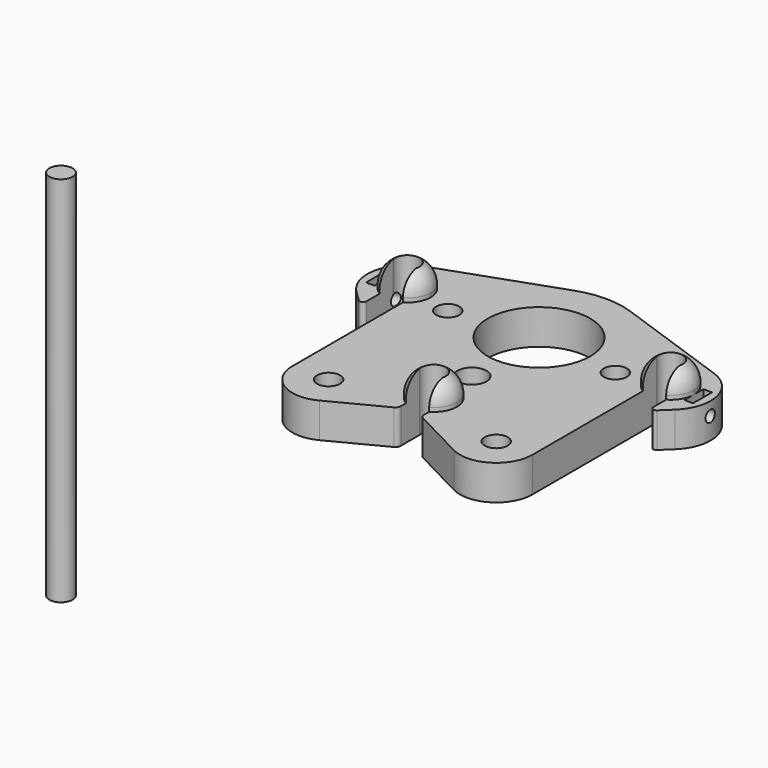
from build123d import *

# Parameters (mm, degrees)
F0_R        = 3.1496
F0_R_2      = 3.9624
F0_R_3      = 16.51
F1_DEPTH    = 9.525
F0_R_4      = 13.97
F2_DEPTH    = 9.525
F5_DEPTH    = 8.636
F6_T1_DEPTH = 2.3368
F6_T3_DEPTH = 2.3368
F7_DEPTH    = 6.35
F8_T2_ANGLE = 359.64
F8_T4_ANGLE = 359.64
F8_T6_ANGLE = 359.64
F10_R       = 1.5875
F11_DEPTH   = 6.35
F9_R        = 1.5875
F12_DEPTH   = 6.35
F13_R       = 3.175
F14_DEPTH   = 50.8


# Not quite as in the source:
# - a fillet or chamfer that OpenCascade refuses, or shapes differently, is made with other operations: its cross-section is extruded or revolved along the edge and cut away or added
# - a feature names something its author has since deleted; it is built from what else it names


with BuildPart() as f1:
    # F0 (on Top) → F1 (new body)
    with BuildSketch(Plane.XY):
        with BuildLine():
            ThreePointArc((-3.175, -0.9069614104), (0, 3.302), (3.175, -0.9069614104))
            Line((3.175, -0.9069614104), (3.175, -7.259066))
            ThreePointArc((3.175, -7.259066), (3.3966960618, -8.05063435), (3.9972840586, -8.6119040308))
            Line((3.9972840586, -8.6119040308), (18.3080023151, -16.0348614764))
            ThreePointArc((18.3080023151, -16.0348614764), (27.9948659534, -15.7070492391), (32.7461149683, -7.259066))
            Line((32.7461149683, -7.259066), (32.7461149683, 35.0139725896))
            ThreePointArc((32.7461149683, 35.0139725896), (35.9211149683, 39.222934), (39.0961149683, 35.0139725896))
            Line((39.0961149683, 35.0139725896), (39.0961149683, 26.0015298192))
            ThreePointArc((39.0961149683, 26.0015298192), (39.6507379199, 25.1601388581), (40.6426301361, 25.3381703138))
            Line((40.6426301361, 25.3381703138), (43.4486259704, 28.0072330887))
            ThreePointArc((43.4486259704, 28.0072330887), (46.6013320921, 38.2063324748), (39.5509253491, 46.2221261931))
            Line((39.5509253491, 46.2221261931), (7.5972775411, 57.4815688228))
            ThreePointArc((7.5972775411, 57.4815688228), (0, 58.780934), (-7.5972775411, 57.4815688228))
            Line((-7.5972775411, 57.4815688228), (-39.5509253491, 46.2221261931))
            ThreePointArc((-39.5509253491, 46.2221261931), (-46.6013320921, 38.2063324748), (-43.4486259704, 28.0072330887))
            Line((-43.4486259704, 28.0072330887), (-40.6507296468, 25.2796426444))
            ThreePointArc((-40.6507296468, 25.2796426444), (-39.6559116262, 25.0916112197), (-39.0961149683, 25.9352025975))
            Line((-39.0961149683, 25.9352025975), (-39.0961149683, 35.0139725896))
            ThreePointArc((-39.0961149683, 35.0139725896), (-35.9211149683, 39.222934), (-32.7461149683, 35.0139725896))
            Line((-32.7461149683, 35.0139725896), (-32.7461149683, -7.259066))
            ThreePointArc((-32.7461149683, -7.259066), (-27.9948659534, -15.7070492391), (-18.3080023151, -16.0348614764))
            Line((-18.3080023151, -16.0348614764), (-3.9972840586, -8.6119040308))
            ThreePointArc((-3.9972840586, -8.6119040308), (-3.3966960618, -8.05063435), (-3.175, -7.259066))
            Line((-3.175, -7.259066), (-3.175, -0.9069614104))
        make_face()
        with Locations((-22.86, -7.259066)):
            Circle(F0_R, mode=Mode.SUBTRACT)
        with Locations((22.86, -7.259066)):
            Circle(F0_R, mode=Mode.SUBTRACT)
        with Locations((0, 13.060934)):
            Circle(F0_R_2, mode=Mode.SUBTRACT)
        with Locations((-22.86, 33.380934)):
            Circle(F0_R, mode=Mode.SUBTRACT)
        with Locations((0, 35.920934)):
            Circle(F0_R_3, mode=Mode.SUBTRACT)
        with Locations((22.86, 33.380934)):
            Circle(F0_R, mode=Mode.SUBTRACT)
    extrude(amount=F1_DEPTH)

    # F0 (on Top) → F2 (join, through all)
    with BuildSketch(Plane.XY):
        with Locations((0, 35.920934)):
            Circle(F0_R_3)
        with Locations((0, 35.920934)):
            Circle(F0_R_4, mode=Mode.SUBTRACT)
    extrude(amount=F2_DEPTH)

    # F4 (on face) → F5 (cut)
    with BuildSketch(Plane.XY.offset(9.525)):
        Polygon((-42.2711149683, 32.695134), (-42.2711149683, 35.920934), (-42.2711149683, 39.146734), (-44.6079149683, 39.146734), (-44.6079149683, 32.695134), align=None)
        Polygon((42.2711149683, 39.146734), (42.2711149683, 35.920934), (42.2711149683, 32.695134), (44.6079149683, 32.695134), (44.6079149683, 39.146734), align=None)
    extrude(amount=-F5_DEPTH, mode=Mode.SUBTRACT)

    # F6: chamfer of 3.175 x 5.499261314 on 4 edges, made by hand

    # F6_s2 → F6_t1 (join)
    with BuildSketch(Plane.YZ.offset(-44.6079149683)):
        Polygon((39.146734, 4.064), (33.647472686, 0.889), (39.146734, 0.889), align=None)
        Polygon((32.695134, 4.064), (38.194395314, 0.889), (32.695134, 0.889), align=None)
    extrude(amount=F6_T1_DEPTH)

    # F6_s4 → F6_t3 (join)
    with BuildSketch(Plane.YZ.offset(42.2711149683)):
        Polygon((39.146734, 4.064), (33.647472686, 0.889), (39.146734, 0.889), align=None)
        Polygon((32.695134, 4.064), (38.194395314, 0.889), (32.695134, 0.889), align=None)
    extrude(amount=F6_T3_DEPTH)

    # F3 (on face) → F7 (join)
    with BuildSketch(Plane.XY.offset(9.525)):
        with BuildLine():
            ThreePointArc((-32.7461149683, 30.421672686), (-30.4218536543, 32.745934), (-29.5711149683, 35.920934))
            ThreePointArc((-29.5711149683, 35.920934), (-39.0961149683, 41.420195314), (-39.0961149683, 30.421672686))
            Line((-39.0961149683, 30.421672686), (-39.0961149683, 35.0139725896))
            ThreePointArc((-39.0961149683, 35.0139725896), (-35.9211149683, 39.222934), (-32.7461149683, 35.0139725896))
            Line((-32.7461149683, 35.0139725896), (-32.7461149683, 30.421672686))
        make_face()
        with BuildLine():
            Line((39.0961149683, 35.0139725896), (39.0961149683, 30.421672686))
            ThreePointArc((39.0961149683, 30.421672686), (41.4203762824, 32.745934), (42.2711149683, 35.920934))
            ThreePointArc((42.2711149683, 35.920934), (32.7461149683, 41.420195314), (32.7461149683, 30.421672686))
            Line((32.7461149683, 30.421672686), (32.7461149683, 35.0139725896))
            ThreePointArc((32.7461149683, 35.0139725896), (35.9211149683, 39.222934), (39.0961149683, 35.0139725896))
        make_face()
        with BuildLine():
            ThreePointArc((6.35, 0), (-3.175, 5.499261314), (-3.175, -5.499261314))
            Line((-3.175, -5.499261314), (-3.175, -0.9069614104))
            ThreePointArc((-3.175, -0.9069614104), (0, 3.302), (3.175, -0.9069614104))
            Line((3.175, -0.9069614104), (3.175, -5.499261314))
            ThreePointArc((3.175, -5.499261314), (5.499261314, -3.175), (6.35, 0))
        make_face()
    extrude(amount=F7_DEPTH)

    # F8: fillet of radius 6.096 on 3 edges, made by hand

    # F8_s1 → F8_t2 (revolve, cut)
    with BuildSketch(Plane(origin=(-35.8079122424, -0.1124942441, 0), x_dir=(0, 0, 1), z_dir=(-0.9999950652, -0.0031415875, 0))):
        with BuildLine():
            ThreePointArc((15.875, 32.7316060627), (13.6437091385, 30.5003152012), (10.5957091385, 29.6836060627))
            Line((10.5957091385, 29.6836060627), (15.875, 29.6836060627))
            Line((15.875, 29.6836060627), (15.875, 32.7316060627))
        make_face()
    revolve(axis=Axis((-35.9211149683, 35.920934, 15.875), (0, 0, 1)), revolution_arc=F8_T2_ANGLE, mode=Mode.SUBTRACT)

    # F8_s3 → F8_t4 (revolve, cut)
    with BuildSketch(Plane(origin=(36.0336086421, 0.1132032926, 0), x_dir=(0, 0, 1), z_dir=(-0.9999950652, -0.0031415875, 0))):
        with BuildLine():
            ThreePointArc((15.875, 32.5059074122), (13.6437091385, 30.2746165507), (10.5957091385, 29.4579074122))
            Line((10.5957091385, 29.4579074122), (15.875, 29.4579074122))
            Line((15.875, 29.4579074122), (15.875, 32.5059074122))
        make_face()
    revolve(axis=Axis((35.9211149683, 35.920934, 15.875), (0, 0, 1)), revolution_arc=F8_T4_ANGLE, mode=Mode.SUBTRACT)

    # F8_s5 → F8_t6 (revolve, cut)
    with BuildSketch(Plane(origin=(0, 0, 0), x_dir=(0, 0, 1), z_dir=(-0.9999950652, -0.0031415875, 0))):
        with BuildLine():
            ThreePointArc((15.875, -3.302), (13.6437091385, -5.5332908615), (10.5957091385, -6.35))
            Line((10.5957091385, -6.35), (15.875, -6.35))
            Line((15.875, -6.35), (15.875, -3.302))
        make_face()
    revolve(axis=Axis((0, 0, 15.875), (0, 0, 1)), revolution_arc=F8_T6_ANGLE, mode=Mode.SUBTRACT)

    # F10 (on face) → F11 (cut, symmetric)
    with BuildSketch(Plane(origin=(44.6079149683, 0, 0), x_dir=(0, -1, 0), z_dir=(-1, 0, 0))):
        with Locations((-35.8627085169, 5.8928)):
            Circle(F10_R)
    extrude(amount=F11_DEPTH, both=True, mode=Mode.SUBTRACT)

    # F9 (on face) → F12 (cut, symmetric)
    with BuildSketch(Plane.YZ.offset(-44.6079149683)):
        with Locations((35.8627085169, 5.8928)):
            Circle(F9_R)
    extrude(amount=F12_DEPTH, both=True, mode=Mode.SUBTRACT)


with BuildPart() as f14:
    # F13 (on Top) → F14 (new body, symmetric)
    with BuildSketch(Plane.XY):
        with Locations((-77.524073422, -30.1994029433)):
            Circle(F13_R)
    extrude(amount=F14_DEPTH, both=True)


solid = Compound([f1.part, f14.part])
